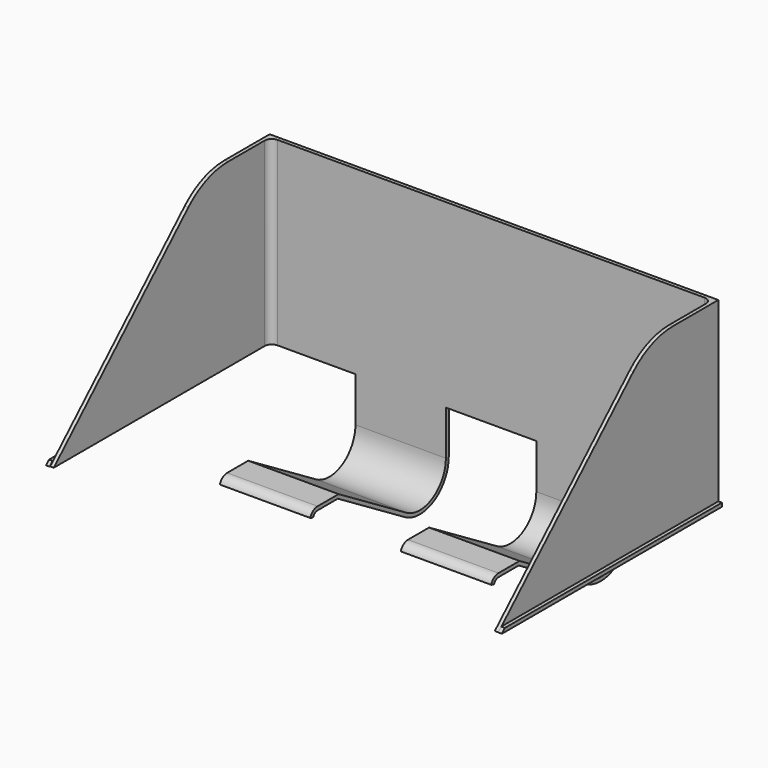
from build123d import *

# Parameters (mm, degrees)
F1_DEPTH  = 50
F3_DEPTH  = 1
F5_DEPTH  = 1
F6_DEPTH  = 1
F7_SIZE   = 0.99999
F9_DEPTH  = 37.5
F10_DEPTH = 12.5
F11_R     = 20


# Not quite as in the source:
# - a fillet or chamfer is up to 0.001 mm smaller than in the source, because OpenCascade refuses the exact size


with BuildPart() as f1:
    # F0 (on Top) → F1 (new body)
    with BuildSketch(Plane.XY):
        with BuildLine():
            Line((-59, 0), (0, 0))
            Line((0, 0), (59, 0))
            ThreePointArc((59, 0), (60.4142135624, -0.5857864376), (61, -2))
            Line((61, -2), (61, -22.5753318518))
            Line((61, -22.5753318518), (62, -22.5753318518))
            Line((62, -22.5753318518), (62, 1))
            Line((62, 1), (0, 1))
            Line((0, 1), (-62, 1))
            Line((-62, 1), (-62, -22.5753318518))
            Line((-62, -22.5753318518), (-61, -22.5753318518))
            Line((-61, -22.5753318518), (-61, -2))
            ThreePointArc((-61, -2), (-60.4142135624, -0.5857864376), (-59, 0))
        make_face()
    extrude(amount=F1_DEPTH)

    # F2 (on face) → F3 (join)
    with BuildSketch(Plane(origin=(-62, 0, 0), x_dir=(0, -1, 0), z_dir=(-1, 0, 0))):
        Polygon((74.8511105776, 0), (22.5753318518, 50), (22.5753318518, 0), align=None)
    extrude(amount=-F3_DEPTH)

    # F4 (on face) → F5 (join)
    with BuildSketch(Plane.YZ.offset(62)):
        Polygon((-22.5753318518, 0), (-22.5753318518, 50), (-74.9809518456, 0), align=None)
    extrude(amount=-F5_DEPTH)

    # F0 (on Top) → F6 (join)
    with BuildSketch(Plane.XY):
        Polygon((62, 1), (62, -22.5753318518), (62, -75), (63, -75), (63, 1), align=None)
        Polygon((-62, -75), (-62, -22.5753318518), (-62, 1), (-63, 1), (-63, -75), align=None)
    extrude(amount=F6_DEPTH)

    # F7 (size 1 in the source; OpenCascade refuses exactly that, so slightly less here)
    f7_edges = [f1.edges().sort_by_distance(p)[0] for p in [
        (62.5, -75, 1),
        (-62.5, -75, 1),
    ]]
    chamfer(f7_edges, length=F7_SIZE)

    # F8 (on Right) → F9 (join, symmetric)
    with BuildSketch(Plane.YZ):
        with BuildLine():
            Line((1, -12.3380962103), (1, 0))
            Line((1, 0), (-6.78e-08, 0))
            Line((-6.78e-08, 0), (-6.78e-08, -12.3380962103))
            ThreePointArc((-6.78e-08, -12.3380962103), (-4.5657106986, -20.1698953121), (-13.6304617639, -20.0555324836))
            Line((-13.6304617639, -20.0555324836), (-37.0563493496, -5.9999999322))
            Line((-37.0563493496, -5.9999999322), (-44.3333333333, -5.9999999322))
            ThreePointArc((-44.3333333333, -5.9999999322), (-45.8844675886, -6.5087526502), (-46.8329720249, -7.8373557287))
            Line((-46.8329720249, -7.8373557287), (-45.8785471313, -8.1358071621))
            ThreePointArc((-45.8785471313, -8.1358071621), (-45.2922055343, -7.3144981402), (-44.3333333333, -7))
            Line((-44.3333333333, -7), (-37.3333333333, -7))
            Line((-37.3333333333, -7), (-14.1449575543, -20.9130254674))
            ThreePointArc((-14.1449575543, -20.9130254674), (-4.0730118502, -21.0400952778), (1, -12.3380962103))
        make_face()
    extrude(amount=F9_DEPTH, both=True)

    # F8 (on Right) → F10 (cut, symmetric)
    with BuildSketch(Plane.YZ):
        with BuildLine():
            Line((1, -12.3380962103), (1, 0))
            Line((1, 0), (-6.78e-08, 0))
            Line((-6.78e-08, 0), (-6.78e-08, -12.3380962103))
            ThreePointArc((-6.78e-08, -12.3380962103), (-4.5657106986, -20.1698953121), (-13.6304617639, -20.0555324836))
            Line((-13.6304617639, -20.0555324836), (-37.0563493496, -5.9999999322))
            Line((-37.0563493496, -5.9999999322), (-44.3333333333, -5.9999999322))
            ThreePointArc((-44.3333333333, -5.9999999322), (-45.8844675886, -6.5087526502), (-46.8329720249, -7.8373557287))
            Line((-46.8329720249, -7.8373557287), (-45.8785471313, -8.1358071621))
            ThreePointArc((-45.8785471313, -8.1358071621), (-45.2922055343, -7.3144981402), (-44.3333333333, -7))
            Line((-44.3333333333, -7), (-37.3333333333, -7))
            Line((-37.3333333333, -7), (-14.1449575543, -20.9130254674))
            ThreePointArc((-14.1449575543, -20.9130254674), (-4.0730118502, -21.0400952778), (1, -12.3380962103))
        make_face()
    extrude(amount=F10_DEPTH, both=True, mode=Mode.SUBTRACT)

    # F11
    f11_edges = [f1.edges().sort_by_distance(p)[0] for p in [
        (-61.5, -22.575332, 50),
        (61.5, -22.575332, 50),
    ]]
    fillet(f11_edges, radius=F11_R)


solid = f1.part
